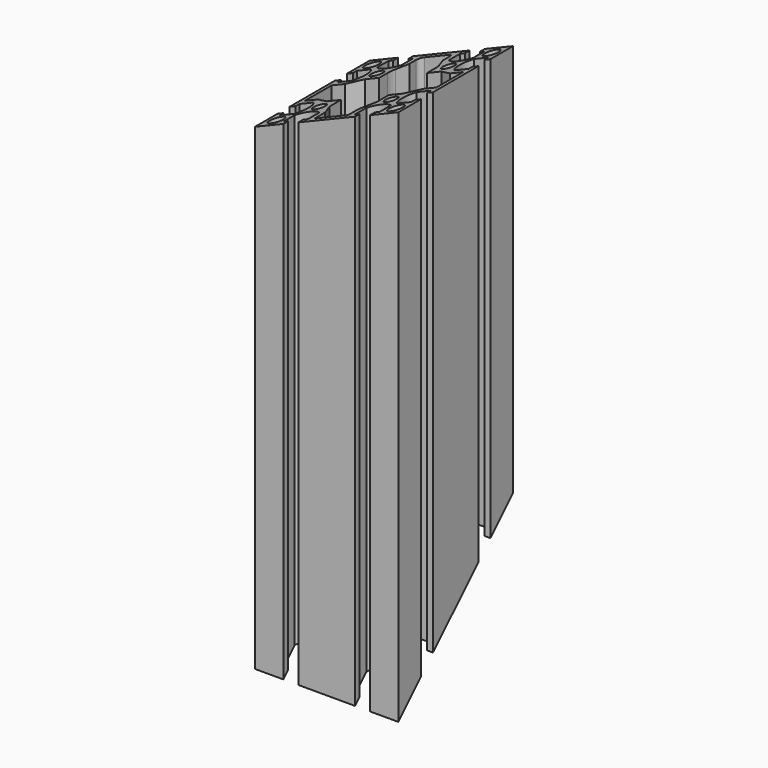
from build123d import *

# Parameters (mm, degrees)
F0_R          = 3
F0_R_2        = 2.5
F1_DEPTH      = 224.6
F2_R          = 2
F3_R          = 7
F6_DEPTH      = 30
F6_DEPTH_BACK = 30
F8_DEPTH      = 30
F8_DEPTH_BACK = 30


# Not quite as in the source:
# - a feature names something its author has since deleted; it is built from what else it names


with BuildPart() as f1:
    # F0 (on Top) → F1 (new body)
    with BuildSketch(Plane.XY):
        with BuildLine():
            Line((18.15, -30), (30, -30))
            Line((30, -30), (30, -18.15))
            Line((30, -18.15), (27.5, -18.15))
            Line((27.5, -18.15), (27.5, -20.15))
            Line((27.5, -20.15), (21.5477069044, -20.15))
            ThreePointArc((21.5477069044, -20.15), (19.5, -15), (21.5477069044, -9.85))
            Line((21.5477069044, -9.85), (27.5, -9.85))
            Line((27.5, -9.85), (27.5, -11.85))
            Line((27.5, -11.85), (30, -11.85))
            Line((30, -11.85), (30, 11.85))
            Line((30, 11.85), (27.5, 11.85))
            Line((27.5, 11.85), (27.5, 9.85))
            Line((27.5, 9.85), (21.5477069044, 9.85))
            ThreePointArc((21.5477069044, 9.85), (19.5, 15), (21.5477069044, 20.15))
            Line((21.5477069044, 20.15), (27.5, 20.15))
            Line((27.5, 20.15), (27.5, 18.15))
            Line((27.5, 18.15), (30, 18.15))
            Line((30, 18.15), (30, 30))
            Line((30, 30), (18.15, 30))
            Line((18.15, 30), (18.15, 27.5))
            Line((18.15, 27.5), (20.15, 27.5))
            Line((20.15, 27.5), (20.15, 21.5477069044))
            ThreePointArc((20.15, 21.5477069044), (15, 19.5), (9.85, 21.5477069044))
            Line((9.85, 21.5477069044), (9.85, 27.5))
            Line((9.85, 27.5), (11.85, 27.5))
            Line((11.85, 27.5), (11.85, 30))
            Line((11.85, 30), (-11.85, 30))
            Line((-11.85, 30), (-11.85, 27.5))
            Line((-11.85, 27.5), (-9.85, 27.5))
            Line((-9.85, 27.5), (-9.85, 21.5477069044))
            ThreePointArc((-9.85, 21.5477069044), (-15, 19.5), (-20.15, 21.5477069044))
            Line((-20.15, 21.5477069044), (-20.15, 27.5))
            Line((-20.15, 27.5), (-18.15, 27.5))
            Line((-18.15, 27.5), (-18.15, 30))
            Line((-18.15, 30), (-30, 30))
            Line((-30, 30), (-30, 18.15))
            Line((-30, 18.15), (-27.5, 18.15))
            Line((-27.5, 18.15), (-27.5, 20.15))
            Line((-27.5, 20.15), (-21.5477069044, 20.15))
            ThreePointArc((-21.5477069044, 20.15), (-19.5, 15), (-21.5477069044, 9.85))
            Line((-21.5477069044, 9.85), (-27.5, 9.85))
            Line((-27.5, 9.85), (-27.5, 11.85))
            Line((-27.5, 11.85), (-30, 11.85))
            Line((-30, 11.85), (-30, -11.85))
            Line((-30, -11.85), (-27.5, -11.85))
            Line((-27.5, -11.85), (-27.5, -9.85))
            Line((-27.5, -9.85), (-21.5477069044, -9.85))
            ThreePointArc((-21.5477069044, -9.85), (-19.5, -15), (-21.5477069044, -20.15))
            Line((-21.5477069044, -20.15), (-27.5, -20.15))
            Line((-27.5, -20.15), (-27.5, -18.15))
            Line((-27.5, -18.15), (-30, -18.15))
            Line((-30, -18.15), (-30, -30))
            Line((-30, -30), (-18.15, -30))
            Line((-18.15, -30), (-18.15, -27.5))
            Line((-18.15, -27.5), (-20.15, -27.5))
            Line((-20.15, -27.5), (-20.15, -21.5477069044))
            ThreePointArc((-20.15, -21.5477069044), (-15, -19.5), (-9.85, -21.5477069044))
            Line((-9.85, -21.5477069044), (-9.85, -27.5))
            Line((-9.85, -27.5), (-11.85, -27.5))
            Line((-11.85, -27.5), (-11.85, -30))
            Line((-11.85, -30), (11.85, -30))
            Line((11.85, -30), (11.85, -27.5))
            Line((11.85, -27.5), (9.85, -27.5))
            Line((9.85, -27.5), (9.85, -21.5477069044))
            ThreePointArc((9.85, -21.5477069044), (15, -19.5), (20.15, -21.5477069044))
            Line((20.15, -21.5477069044), (20.15, -27.5))
            Line((20.15, -27.5), (18.15, -27.5))
            Line((18.15, -27.5), (18.15, -30))
        make_face()
        with Locations((-25, -25)):
            Circle(F0_R, mode=Mode.SUBTRACT)
        with Locations((-15, -15)):
            Circle(F0_R_2, mode=Mode.SUBTRACT)
        with Locations((25, -25)):
            Circle(F0_R, mode=Mode.SUBTRACT)
        with Locations((15, -15)):
            Circle(F0_R_2, mode=Mode.SUBTRACT)
        with Locations((-25, 25)):
            Circle(F0_R, mode=Mode.SUBTRACT)
        with Locations((-15, 15)):
            Circle(F0_R_2, mode=Mode.SUBTRACT)
        Polygon((-7, 22), (-7, 27.5), (0, 27.5), (7, 27.5), (7, 22), (10, 16), (10, 10), (16, 10), (22, 7), (27.5, 7), (27.5, 0), (27.5, -7), (22, -7), (16, -10), (10, -10), (10, -16), (7, -22), (7, -27.5), (0, -27.5), (-7, -27.5), (-7, -22), (-10, -16), (-10, -10), (-16, -10), (-22, -7), (-27.5, -7), (-27.5, 0), (-27.5, 7), (-22, 7), (-16, 10), (-10, 10), (-10, 16), align=None, mode=Mode.SUBTRACT)
        with Locations((15, 15)):
            Circle(F0_R_2, mode=Mode.SUBTRACT)
        with Locations((25, 25)):
            Circle(F0_R, mode=Mode.SUBTRACT)
    extrude(amount=F1_DEPTH)

    # F2
    f2_edges = [f1.edges().sort_by_distance(p)[0] for p in [
        (-7, 27.5, 112.3),
        (7, 27.5, 112.3),
    ]]
    fillet(f2_edges, radius=F2_R)

    # F3
    f3_edges = [f1.edges().sort_by_distance(p)[0] for p in [
        (-10, 16, 112.3),
        (10, 16, 112.3),
    ]]
    fillet(f3_edges, radius=F3_R)

    # F5 (on Right) → F6 (cut, two sides)
    with BuildSketch(Plane.YZ) as f6_sk:
        Polygon((70.3932136338, -100.3932136338), (211.6390804038, 40.8526531362), (111.24586677, 141.24586677), (-30, 0), align=None)
    extrude(amount=-F6_DEPTH, mode=Mode.SUBTRACT)
    extrude(f6_sk.sketch, amount=F6_DEPTH_BACK, mode=Mode.SUBTRACT)

    # F7 (on Front) → F8 (cut, two sides)
    with BuildSketch(Plane.XZ) as f8_sk:
        Polygon((-32.0951359741, 374.5109194261), (-136.0873846676, 331.4359196356), (-73.9922486935, 181.5250002095), (30, 224.6), align=None)
    extrude(amount=F8_DEPTH, mode=Mode.SUBTRACT)
    extrude(f8_sk.sketch, amount=-F8_DEPTH_BACK, mode=Mode.SUBTRACT)


solid = f1.part
